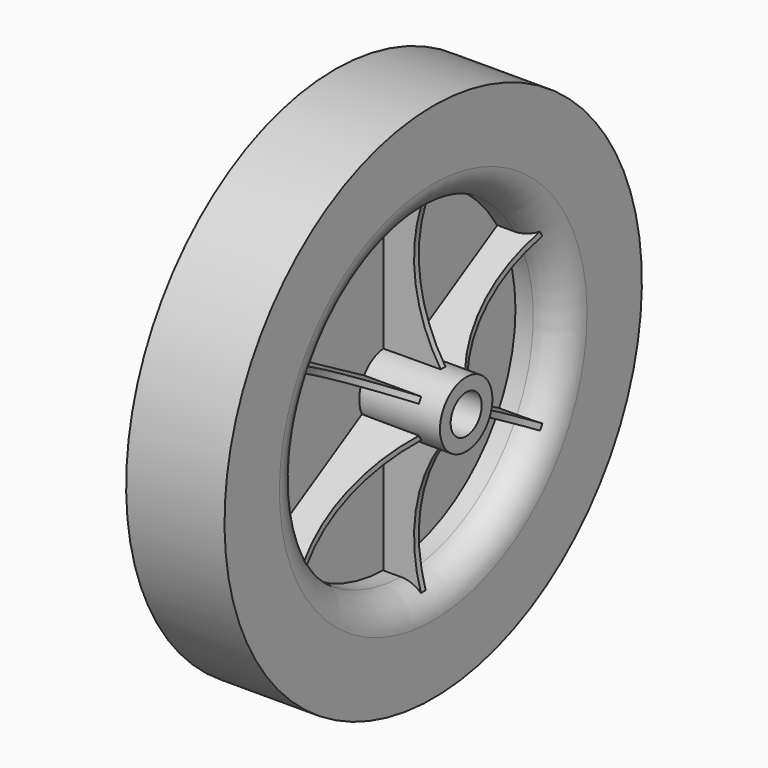
from build123d import *

# Parameters (mm, degrees)
F3_R            = 10
F5_DEPTH        = 1
F5_COPIES_COUNT = 6


# Not quite as in the source:
# - a pattern or mirror of a feature is missing from the dataset's text; its kind, count and spacing are read off the source's solid


with BuildPart() as f2:
    # F1 (on Front) → F2 (revolve)
    with BuildSketch(Plane.XZ):
        Polygon((17.9380366504, 54.5), (17.9380366504, 87.5), (-15.0619633496, 87.5), (-15.0619633496, 54.5), (-1.0619633496, 54.5), (-1.0619633496, 15), (-9, 15), (-9, 6.5), (29, 6.5), (29, 11), (1.9380366504, 11), (1.9380366504, 54.5), align=None)
    revolve(axis=Axis((-1.7091594636, 0, 0), (1, 0, 0)))

    # F3
    f3_edges = [f2.edges().sort_by_distance(p)[0] for p in [
        (17.938037, 0, -54.5),
        (-15.061963, 0, -54.5),
    ]]
    fillet(f3_edges, radius=F3_R)

    # F4 (on Front) → F5 (join, symmetric)
    with BuildSketch(Plane.XZ):
        with BuildLine():
            ThreePointArc((21.256512031, 11.1461849883), (12.8744275284, 33.3890012192), (14.6401561797, 57.0931024849))
            Line((14.6401561797, 57.0931024849), (2.0852813032, 57.0931024849))
            Line((2.0852813032, 57.0931024849), (2.0852813032, 11.0397199169))
            Line((2.0852813032, 11.0397199169), (21.256512031, 11.1461849883))
        make_face()
    f5 = extrude(amount=F5_DEPTH, both=True)

    # F5_copies: F5 ×6 about axis
    f5_copies_axis = Axis((0, 0, 0), (1, 0, 0))
    for i in range(1, F5_COPIES_COUNT):
        add(f5.rotate(f5_copies_axis, i * 360 / F5_COPIES_COUNT))


solid = f2.part
